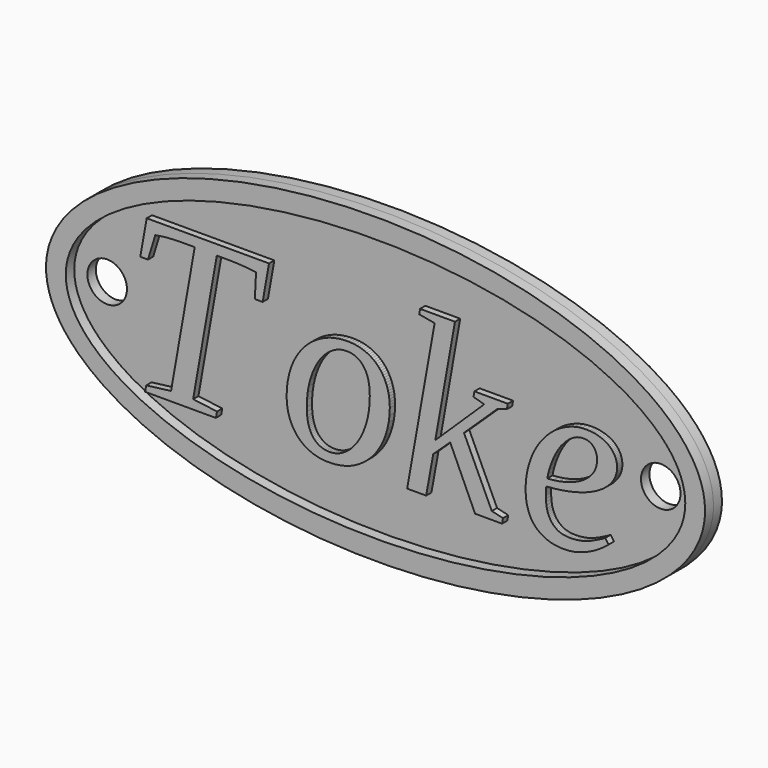
from build123d import *

# Parameters (mm, degrees)
F0_R     = 3
F1_DEPTH = 1.6
F2_DEPTH = 1.6
F3_DEPTH = 1


# Not quite as in the source:
# - a feature names something its author has since deleted; it is built from what else it names


with BuildPart() as f1:
    # F0 (on Front) → F1 (new body)
    with BuildSketch(Plane.XZ):
        with BuildLine():
            add(Edge.make_bspline(
                [(50, 0), (50, 39.8371685741), (-25, 19.918584287), (-100, 0), (-25, -19.918584287), (50, -39.8371685741), (50, 0)],
                knots=[0, 0, 0, 2.0943951024, 2.0943951024, 4.1887902048, 4.1887902048, 6.2831853072, 6.2831853072, 6.2831853072], degree=2, weights=[1, 0.5, 1, 0.5, 1, 0.5, 1]))
        make_face()
        with BuildLine():
            add(Edge.make_bspline(
                [(47, 0), (47, 34.6410161514), (-23.5, 17.3205080757), (-94, 0), (-23.5, -17.3205080757), (47, -34.6410161514), (47, 0)],
                knots=[0, 0, 0, 2.0943951024, 2.0943951024, 4.1887902048, 4.1887902048, 6.2831853072, 6.2831853072, 6.2831853072], degree=2, weights=[1, 0.5, 1, 0.5, 1, 0.5, 1]))
        make_face(mode=Mode.SUBTRACT)
        with BuildLine():
            add(Edge.make_bspline(
                [(47, 0), (47, 34.6410161514), (-23.5, 17.3205080757), (-94, 0), (-23.5, -17.3205080757), (47, -34.6410161514), (47, 0)],
                knots=[0, 0, 0, 2.0943951024, 2.0943951024, 4.1887902048, 4.1887902048, 6.2831853072, 6.2831853072, 6.2831853072], degree=2, weights=[1, 0.5, 1, 0.5, 1, 0.5, 1]))
        make_face()
        Polygon((-24.7064, -12.153), (-35.4455, -12.153), (-35.272, -11.2335), (-31.5072, -10.7651), (-27.916, 9.6201), (-28.8008, 9.6201), (-29.3451, 9.6179), (-29.8504, 9.6114), (-30.3166, 9.6006), (-30.5351, 9.5935), (-30.7439, 9.5854), (-31.1375, 9.5745), (-31.5029, 9.5594), (-31.8401, 9.5398), (-31.9982, 9.5284), (-32.1491, 9.516), (-32.4332, 9.4889), (-32.6956, 9.4596), (-32.8187, 9.4441), (-32.9364, 9.4281), (-33.0486, 9.4116), (-33.1554, 9.3945), (-33.3582, 9.3674), (-33.5501, 9.3382), (-33.7312, 9.3067), (-33.9014, 9.2731), (-35.0117, 5.6471), (-36.1741, 5.6471), (-35.2026, 11.1121), (-16.6391, 11.1121), (-17.6106, 5.6471), (-18.7904, 5.6471), (-18.6169, 9.2731), (-18.6952, 9.2881), (-18.7784, 9.3029), (-18.8665, 9.3174), (-18.9595, 9.3316), (-19.0574, 9.3456), (-19.1601, 9.3593), (-19.2677, 9.3727), (-19.4976, 9.3987), (-19.747, 9.4237), (-20.0159, 9.4475), (-20.3043, 9.4703), (-20.4559, 9.4813), (-20.7763, 9.5057), (-21.1216, 9.5268), (-21.4919, 9.5447), (-21.8872, 9.5594), (-22.3073, 9.5707), (-22.7525, 9.5789), (-23.2225, 9.5837), (-23.7175, 9.5854), (-24.5676, 9.5854), (-28.1589, -10.7651), (-24.5329, -11.2335), align=None, mode=Mode.SUBTRACT)
        Polygon((-7.0857, -12.487), (-7.6167, -12.5), (-7.9645, -12.4927), (-8.3052, -12.4707), (-8.6389, -12.4341), (-8.9656, -12.3829), (-9.2852, -12.317), (-9.5977, -12.2365), (-9.9033, -12.1413), (-10.2017, -12.0316), (-10.4874, -11.9079), (-10.7634, -11.7713), (-11.0296, -11.6217), (-11.286, -11.459), (-11.5327, -11.2834), (-11.7696, -11.0947), (-11.9968, -10.893), (-12.2142, -10.6783), (-12.4167, -10.4512), (-12.6078, -10.2121), (-12.7875, -9.9611), (-12.9559, -9.6981), (-13.1128, -9.4232), (-13.2584, -9.1364), (-13.3926, -8.8377), (-13.5154, -8.527), (-13.6211, -8.2053), (-13.7127, -7.8732), (-13.7903, -7.5308), (-13.8537, -7.1782), (-13.903, -6.8152), (-13.9383, -6.4419), (-13.9594, -6.0583), (-13.9665, -5.6645), (-13.9263, -4.6604), (-13.806, -3.678), (-13.6054, -2.7173), (-13.3245, -1.7783), (-13.1513, -1.3212), (-12.9613, -0.8783), (-12.7545, -0.4494), (-12.5308, -0.0347), (-12.2904, 0.366), (-12.0331, 0.7525), (-11.7591, 1.125), (-11.4682, 1.4834), (-11.1567, 1.8298), (-10.8295, 2.1578), (-10.4866, 2.4674), (-10.128, 2.7585), (-9.7536, 3.0312), (-9.3635, 3.2855), (-8.9577, 3.5213), (-8.5362, 3.7387), (-8.1, 3.938), (-7.6503, 4.1107), (-7.187, 4.2568), (-6.7102, 4.3763), (-6.2198, 4.4693), (-5.7159, 4.5357), (-5.1984, 4.5756), (-4.6674, 4.5888), (-4.3198, 4.5815), (-3.9799, 4.5596), (-3.6476, 4.523), (-3.3228, 4.4717), (-3.0056, 4.4059), (-2.6961, 4.3254), (-2.3941, 4.2302), (-2.0997, 4.1204), (-1.8102, 3.9968), (-1.5315, 3.8602), (-1.2637, 3.7105), (-1.0067, 3.5479), (-0.7606, 3.3722), (-0.5253, 3.1836), (-0.3008, 2.9819), (-0.0872, 2.7672), (0.1191, 2.54), (0.3129, 2.3009), (0.4943, 2.0499), (0.6631, 1.787), (0.8196, 1.5121), (0.9635, 1.2253), (1.095, 0.9266), (1.214, 0.6159), (1.3238, 0.2941), (1.4189, -0.0379), (1.4994, -0.3803), (1.5653, -0.733), (1.6165, -1.096), (1.6531, -1.4692), (1.6751, -1.8528), (1.6824, -2.2467), (1.6412, -3.2508), (1.5176, -4.2332), (1.3116, -5.1939), (1.0231, -6.1329), (0.8537, -6.5902), (0.6664, -7.0339), (0.4612, -7.4641), (0.2381, -7.8808), (-0.0029, -8.2839), (-0.2618, -8.6734), (-0.5386, -9.0494), (-0.8332, -9.4118), (-1.1406, -9.7545), (-1.4643, -10.0798), (-1.8042, -10.3877), (-2.1604, -10.6783), (-2.5329, -10.9516), (-2.9216, -11.2075), (-3.3266, -11.446), (-3.7479, -11.6672), (-4.184, -11.8624), (-4.6337, -12.0316), (-5.097, -12.1747), (-5.5739, -12.2918), (-6.0642, -12.3829), (-6.5682, -12.4479), align=None, mode=Mode.SUBTRACT)
        Polygon((36.1689, 1.2212), (36.1741, 1.0323), (36.163, 0.7523), (36.1296, 0.476), (36.074, 0.2036), (35.9962, -0.065), (35.8962, -0.3299), (35.774, -0.5909), (35.6295, -0.8482), (35.4628, -1.1016), (35.2746, -1.3502), (35.0659, -1.5928), (34.8366, -1.8295), (34.5866, -2.0602), (34.3161, -2.2849), (34.025, -2.5037), (33.7132, -2.7165), (33.3809, -2.9233), (33.0323, -3.119), (32.6631, -3.3071), (32.2732, -3.4877), (31.8628, -3.6606), (31.4318, -3.826), (30.9802, -3.9838), (30.0152, -4.2765), (28.9807, -4.5227), (27.8725, -4.7233), (26.6906, -4.8783), (25.435, -4.9878), (25.4328, -5.008), (25.4304, -5.0296), (25.4279, -5.0525), (25.4252, -5.0768), (25.4225, -5.1024), (25.4195, -5.1293), (25.4165, -5.1577), (25.4133, -5.1874), (25.4065, -5.2508), (25.3992, -5.3196), (25.3914, -5.3939), (25.383, -5.4736), (25.3789, -5.5579), (25.3724, -5.7379), (25.368, -5.9331), (25.3659, -6.1434), (25.3656, -6.2543), (25.3754, -6.6761), (25.4046, -7.0914), (25.4534, -7.5002), (25.5217, -7.9025), (25.5689, -8.0993), (25.6237, -8.2907), (25.686, -8.4766), (25.756, -8.6572), (25.8335, -8.8323), (25.9186, -9.002), (26.0113, -9.1662), (26.1116, -9.3251), (26.2203, -9.4774), (26.3382, -9.6222), (26.4654, -9.7594), (26.6017, -9.8889), (26.7473, -10.0109), (26.9021, -10.1253), (27.0661, -10.2321), (27.2393, -10.3313), (27.4231, -10.4167), (27.6188, -10.4907), (27.8265, -10.5534), (28.046, -10.6046), (28.2775, -10.6444), (28.521, -10.6729), (28.7763, -10.69), (29.0436, -10.6957), (29.4302, -10.6875), (29.8091, -10.6631), (30.1805, -10.6225), (30.5443, -10.5656), (30.9005, -10.4924), (31.2491, -10.4029), (31.5901, -10.2972), (31.9235, -10.1752), (32.572, -9.8976), (33.8038, -9.2904), (34.3871, -8.9608), (34.8902, -9.6894), (34.6007, -9.9258), (34.2874, -10.1665), (33.9501, -10.4116), (33.5891, -10.661), (33.2074, -10.9071), (32.8083, -11.1424), (31.9582, -11.5805), (31.518, -11.7713), (31.0648, -11.9448), (30.5985, -12.101), (30.1192, -12.2397), (29.6313, -12.3536), (29.139, -12.4349), (28.6424, -12.4837), (28.1415, -12.5), (27.7787, -12.4935), (27.428, -12.474), (27.0891, -12.4414), (26.7622, -12.3959), (26.4472, -12.3373), (26.1441, -12.2658), (25.853, -12.1812), (25.5738, -12.0836), (25.3062, -11.9697), (25.0501, -11.8451), (24.8053, -11.7095), (24.5719, -11.5631), (24.3499, -11.4059), (24.1392, -11.2378), (23.94, -11.0589), (23.7521, -10.8692), (23.5757, -10.6686), (23.4106, -10.4571), (23.2569, -10.2348), (23.1146, -10.0017), (22.9836, -9.7577), (22.8641, -9.5029), (22.7559, -9.2373), (22.6591, -8.9608), (22.5738, -8.6745), (22.4998, -8.3796), (22.4371, -8.076), (22.3859, -7.7637), (22.3461, -7.4427), (22.3005, -6.7748), (22.2948, -6.4278), (22.3165, -5.6645), (22.3816, -4.9184), (22.49, -4.1898), (22.6418, -3.4785), (22.8326, -2.7802), (23.0582, -2.1079), (23.3184, -1.4616), (23.6133, -0.8414), (23.9408, -0.2407), (24.2986, 0.3297), (24.6868, 0.8696), (25.1054, 1.3793), (25.5478, 1.864), (26.0075, 2.3118), (26.4846, 2.7227), (26.9791, 3.0968), (27.4974, 3.4319), (28.0287, 3.7257), (28.573, 3.9784), (29.1303, 4.1898), (29.705, 4.3644), (30.2841, 4.4891), (30.8674, 4.5639), (31.4551, 4.5888), (31.9951, 4.5715), (32.2537, 4.5498), (32.5047, 4.5194), (32.7482, 4.4804), (32.984, 4.4327), (33.2123, 4.3763), (33.4329, 4.3113), (33.6498, 4.2427), (33.858, 4.167), (34.0575, 4.0844), (34.2483, 3.9946), (34.4305, 3.8979), (34.604, 3.794), (34.7688, 3.6832), (34.9249, 3.5653), (35.0721, 3.4452), (35.2101, 3.3191), (35.3389, 3.1871), (35.4584, 3.0491), (35.5687, 2.9052), (35.6699, 2.7553), (35.7618, 2.5994), (35.8444, 2.4376), (35.9217, 2.2752), (35.9887, 2.109), (36.0453, 1.939), (36.0917, 1.7653), (36.1277, 1.5877), (36.1535, 1.4064), align=None, mode=Mode.SUBTRACT)
        with Locations((-42, 0)):
            Circle(F0_R, mode=Mode.SUBTRACT)
        Polygon((4.3203, -12.153), (8.4841, 11.3029), (6.142, 11.7193), (6.2808, 12.5), (11.5722, 12.5), (8.5882, -4.2939), (16.0136, 2.906), (14.3828, 3.3744), (14.5216, 4.1551), (19.5875, 4.1551), (19.4487, 3.3744), (18.0434, 2.9754), (12.9428, -1.8997), (17.1586, -10.9733), (18.8588, -11.3723), (18.72, -12.153), (14.6257, -12.153), (10.8436, -3.8428), (8.2759, -6.2543), (7.2003, -12.153), align=None, mode=Mode.SUBTRACT)
        with Locations((42, 0)):
            Circle(F0_R, mode=Mode.SUBTRACT)
        Polygon((-7.9645, -12.4927), (-7.6167, -12.5), (-7.0857, -12.487), (-6.5682, -12.4479), (-6.0642, -12.3829), (-5.5739, -12.2918), (-5.097, -12.1747), (-4.6337, -12.0316), (-4.184, -11.8624), (-3.7479, -11.6672), (-3.3266, -11.446), (-2.9216, -11.2075), (-2.5329, -10.9516), (-2.1604, -10.6783), (-1.8042, -10.3877), (-1.4643, -10.0798), (-1.1406, -9.7545), (-0.8332, -9.4118), (-0.5386, -9.0494), (-0.2618, -8.6734), (-0.0029, -8.2839), (0.2381, -7.8808), (0.4612, -7.4641), (0.6664, -7.0339), (0.8537, -6.5902), (1.0231, -6.1329), (1.3116, -5.1939), (1.5176, -4.2332), (1.6412, -3.2508), (1.6824, -2.2467), (1.6751, -1.8528), (1.6531, -1.4692), (1.6165, -1.096), (1.5653, -0.733), (1.4994, -0.3803), (1.4189, -0.0379), (1.3238, 0.2941), (1.214, 0.6159), (1.095, 0.9266), (0.9635, 1.2253), (0.8196, 1.5121), (0.6631, 1.787), (0.4943, 2.0499), (0.3129, 2.3009), (0.1191, 2.54), (-0.0872, 2.7672), (-0.3008, 2.9819), (-0.5253, 3.1836), (-0.7606, 3.3722), (-1.0067, 3.5479), (-1.2637, 3.7105), (-1.5315, 3.8602), (-1.8102, 3.9968), (-2.0997, 4.1204), (-2.3941, 4.2302), (-2.6961, 4.3254), (-3.0056, 4.4059), (-3.3228, 4.4717), (-3.6476, 4.523), (-3.9799, 4.5596), (-4.3198, 4.5815), (-4.6674, 4.5888), (-5.1984, 4.5756), (-5.7159, 4.5357), (-6.2198, 4.4693), (-6.7102, 4.3763), (-7.187, 4.2568), (-7.6503, 4.1107), (-8.1, 3.938), (-8.5362, 3.7387), (-8.9577, 3.5213), (-9.3635, 3.2855), (-9.7536, 3.0312), (-10.128, 2.7585), (-10.4866, 2.4674), (-10.8295, 2.1578), (-11.1567, 1.8298), (-11.4682, 1.4834), (-11.7591, 1.125), (-12.0331, 0.7525), (-12.2904, 0.366), (-12.5308, -0.0347), (-12.7545, -0.4494), (-12.9613, -0.8783), (-13.1513, -1.3212), (-13.3245, -1.7783), (-13.6054, -2.7173), (-13.806, -3.678), (-13.9263, -4.6604), (-13.9665, -5.6645), (-13.9594, -6.0583), (-13.9383, -6.4419), (-13.903, -6.8152), (-13.8537, -7.1782), (-13.7903, -7.5308), (-13.7127, -7.8732), (-13.6211, -8.2053), (-13.5154, -8.527), (-13.3926, -8.8377), (-13.2584, -9.1364), (-13.1128, -9.4232), (-12.9559, -9.6981), (-12.7875, -9.9611), (-12.6078, -10.2121), (-12.4167, -10.4512), (-12.2142, -10.6783), (-11.9968, -10.893), (-11.7696, -11.0947), (-11.5327, -11.2834), (-11.286, -11.459), (-11.0296, -11.6217), (-10.7634, -11.7713), (-10.4874, -11.9079), (-10.2017, -12.0316), (-9.9033, -12.1413), (-9.5977, -12.2365), (-9.2852, -12.317), (-8.9656, -12.3829), (-8.6389, -12.4341), (-8.3052, -12.4707), align=None)
        Polygon((-10.8989, -6.8228), (-10.913, -6.2543), (-10.8816, -5.2427), (-10.7872, -4.2722), (-10.63, -3.3429), (-10.4099, -2.4549), (-10.279, -2.0247), (-9.9862, -1.2114), (-9.8244, -0.8284), (-9.6522, -0.4611), (-9.4698, -0.1095), (-9.2771, 0.2264), (-9.074, 0.5465), (-8.8618, 0.8545), (-8.6414, 1.1451), (-8.4129, 1.4183), (-8.1762, 1.6742), (-7.9314, 1.9128), (-7.6785, 2.134), (-7.4175, 2.3378), (-7.1483, 2.5243), (-6.8737, 2.691), (-6.5964, 2.8355), (-6.3163, 2.9578), (-6.0336, 3.0578), (-5.7482, 3.1356), (-5.46, 3.1912), (-5.1691, 3.2245), (-4.8755, 3.2356), (-4.6661, 3.2307), (-4.463, 3.2161), (-4.266, 3.1917), (-4.0753, 3.1575), (-3.8909, 3.1136), (-3.7126, 3.06), (-3.5406, 2.9965), (-3.3749, 2.9233), (-3.2153, 2.8404), (-3.062, 2.7477), (-2.915, 2.6452), (-2.7741, 2.533), (-2.6396, 2.411), (-2.5112, 2.2793), (-2.3891, 2.1377), (-2.2732, 1.9865), (-2.1618, 1.828), (-2.0577, 1.6604), (-1.9607, 1.4837), (-1.8709, 1.2979), (-1.7883, 1.1031), (-1.7129, 0.8992), (-1.6446, 0.6862), (-1.5836, 0.4641), (-1.5297, 0.2329), (-1.483, -0.0073), (-1.4435, -0.2566), (-1.4112, -0.515), (-1.3681, -1.0591), (-1.3537, -1.6395), (-1.3862, -2.636), (-1.4838, -3.5956), (-1.6465, -4.5183), (-1.8742, -5.4042), (-2.0054, -5.8266), (-2.3003, -6.629), (-2.6386, -7.375), (-2.824, -7.7268), (-3.0203, -8.0646), (-3.2274, -8.3883), (-3.4399, -8.6924), (-3.6611, -8.9803), (-3.891, -9.2519), (-4.1295, -9.5073), (-4.3768, -9.7464), (-4.6327, -9.9692), (-4.8972, -10.1757), (-5.1705, -10.366), (-5.4454, -10.5328), (-5.7235, -10.6772), (-6.0049, -10.7995), (-6.2895, -10.8995), (-6.5774, -10.9773), (-6.8685, -11.0329), (-7.1629, -11.0662), (-7.4606, -11.0774), (-7.6616, -11.0725), (-7.8571, -11.0581), (-8.0471, -11.0341), (-8.2315, -11.0004), (-8.4104, -10.9571), (-8.5836, -10.9041), (-8.7514, -10.8416), (-8.9135, -10.7694), (-9.0702, -10.6876), (-9.2212, -10.5962), (-9.3667, -10.4951), (-9.5067, -10.3845), (-9.6411, -10.2642), (-9.7699, -10.1343), (-9.8932, -9.9947), (-10.0109, -9.8456), (-10.1201, -9.6852), (-10.2223, -9.5162), (-10.3175, -9.3387), (-10.4056, -9.1527), (-10.4866, -8.9581), (-10.5606, -8.755), (-10.6276, -8.5434), (-10.6875, -8.3232), (-10.7403, -8.0945), (-10.7862, -7.8572), (-10.8249, -7.6114), (-10.8566, -7.3571), align=None, mode=Mode.SUBTRACT)
        Polygon((36.163, 0.7523), (36.1741, 1.0323), (36.1689, 1.2212), (36.1535, 1.4064), (36.1277, 1.5877), (36.0917, 1.7653), (36.0453, 1.939), (35.9887, 2.109), (35.9217, 2.2752), (35.8444, 2.4376), (35.7618, 2.5994), (35.6699, 2.7553), (35.5687, 2.9052), (35.4584, 3.0491), (35.3389, 3.1871), (35.2101, 3.3191), (35.0721, 3.4452), (34.9249, 3.5653), (34.7688, 3.6832), (34.604, 3.794), (34.4305, 3.8979), (34.2483, 3.9946), (34.0575, 4.0844), (33.858, 4.167), (33.6498, 4.2427), (33.4329, 4.3113), (33.2123, 4.3763), (32.984, 4.4327), (32.7482, 4.4804), (32.5047, 4.5194), (32.2537, 4.5498), (31.9951, 4.5715), (31.4551, 4.5888), (30.8674, 4.5639), (30.2841, 4.4891), (29.705, 4.3644), (29.1303, 4.1898), (28.573, 3.9784), (28.0287, 3.7257), (27.4974, 3.4319), (26.9791, 3.0968), (26.4846, 2.7227), (26.0075, 2.3118), (25.5478, 1.864), (25.1054, 1.3793), (24.6868, 0.8696), (24.2986, 0.3297), (23.9408, -0.2407), (23.6133, -0.8414), (23.3184, -1.4616), (23.0582, -2.1079), (22.8326, -2.7802), (22.6418, -3.4785), (22.49, -4.1898), (22.3816, -4.9184), (22.3165, -5.6645), (22.2948, -6.4278), (22.3005, -6.7748), (22.3461, -7.4427), (22.3859, -7.7637), (22.4371, -8.076), (22.4998, -8.3796), (22.5738, -8.6745), (22.6591, -8.9608), (22.7559, -9.2373), (22.8641, -9.5029), (22.9836, -9.7577), (23.1146, -10.0017), (23.2569, -10.2348), (23.4106, -10.4571), (23.5757, -10.6686), (23.7521, -10.8692), (23.94, -11.0589), (24.1392, -11.2378), (24.3499, -11.4059), (24.5719, -11.5631), (24.8053, -11.7095), (25.0501, -11.8451), (25.3062, -11.9697), (25.5738, -12.0836), (25.853, -12.1812), (26.1441, -12.2658), (26.4472, -12.3373), (26.7622, -12.3959), (27.0891, -12.4414), (27.428, -12.474), (27.7787, -12.4935), (28.1415, -12.5), (28.6424, -12.4837), (29.139, -12.4349), (29.6313, -12.3536), (30.1192, -12.2397), (30.5985, -12.101), (31.0648, -11.9448), (31.518, -11.7713), (31.9582, -11.5805), (32.8083, -11.1424), (33.2074, -10.9071), (33.5891, -10.661), (33.9501, -10.4116), (34.2874, -10.1665), (34.6007, -9.9258), (34.8902, -9.6894), (34.3871, -8.9608), (33.8038, -9.2904), (32.572, -9.8976), (31.9235, -10.1752), (31.5901, -10.2972), (31.2491, -10.4029), (30.9005, -10.4924), (30.5443, -10.5656), (30.1805, -10.6225), (29.8091, -10.6631), (29.4302, -10.6875), (29.0436, -10.6957), (28.7763, -10.69), (28.521, -10.6729), (28.2775, -10.6444), (28.046, -10.6046), (27.8265, -10.5534), (27.6188, -10.4907), (27.4231, -10.4167), (27.2393, -10.3313), (27.0661, -10.2321), (26.9021, -10.1253), (26.7473, -10.0109), (26.6017, -9.8889), (26.4654, -9.7594), (26.3382, -9.6222), (26.2203, -9.4774), (26.1116, -9.3251), (26.0113, -9.1662), (25.9186, -9.002), (25.8335, -8.8323), (25.756, -8.6572), (25.686, -8.4766), (25.6237, -8.2907), (25.5689, -8.0993), (25.5217, -7.9025), (25.4534, -7.5002), (25.4046, -7.0914), (25.3754, -6.6761), (25.3656, -6.2543), (25.3659, -6.1434), (25.368, -5.9331), (25.3724, -5.7379), (25.3789, -5.5579), (25.383, -5.4736), (25.3914, -5.3939), (25.3992, -5.3196), (25.4065, -5.2508), (25.4133, -5.1874), (25.4165, -5.1577), (25.4195, -5.1293), (25.4225, -5.1024), (25.4252, -5.0768), (25.4279, -5.0525), (25.4304, -5.0296), (25.4328, -5.008), (25.435, -4.9878), (26.6906, -4.8783), (27.8725, -4.7233), (28.9807, -4.5227), (30.0152, -4.2765), (30.9802, -3.9838), (31.4318, -3.826), (31.8628, -3.6606), (32.2732, -3.4877), (32.6631, -3.3071), (33.0323, -3.119), (33.3809, -2.9233), (33.7132, -2.7165), (34.025, -2.5037), (34.3161, -2.2849), (34.5866, -2.0602), (34.8366, -1.8295), (35.0659, -1.5928), (35.2746, -1.3502), (35.4628, -1.1016), (35.6295, -0.8482), (35.774, -0.5909), (35.8962, -0.3299), (35.9962, -0.065), (36.074, 0.2036), (36.1296, 0.476), align=None)
        Polygon((26.49, -3.8059), (25.5738, -3.8948), (25.7039, -3.2692), (25.8687, -2.6414), (26.0682, -2.0114), (26.3025, -1.3792), (26.567, -0.7536), (26.8576, -0.1605), (27.1742, 0.4001), (27.5169, 0.9282), (27.7018, 1.1781), (28.0878, 1.6422), (28.2889, 1.8564), (28.4955, 2.0586), (28.7075, 2.2489), (28.9249, 2.4273), (29.1477, 2.5937), (29.3751, 2.7482), (29.6064, 2.8821), (29.8414, 2.9954), (30.0802, 3.0882), (30.3228, 3.1603), (30.5692, 3.2118), (30.8194, 3.2427), (31.0734, 3.253), (31.1973, 3.2505), (31.3174, 3.2432), (31.4337, 3.231), (31.5462, 3.2139), (31.6549, 3.192), (31.7598, 3.1651), (31.8609, 3.1334), (31.9582, 3.0968), (32.0518, 3.0553), (32.1415, 3.009), (32.2274, 2.9578), (32.3096, 2.9016), (32.3879, 2.8407), (32.4625, 2.7748), (32.5332, 2.704), (32.6002, 2.6284), (32.6653, 2.549), (32.7262, 2.4668), (32.7829, 2.382), (32.8355, 2.2944), (32.8838, 2.2042), (32.9279, 2.1112), (32.9678, 2.0155), (33.0035, 1.9171), (33.035, 1.816), (33.0624, 1.7122), (33.0855, 1.6056), (33.1044, 1.4964), (33.1191, 1.3844), (33.1296, 1.2698), (33.138, 1.0323), (33.1307, 0.8119), (33.1087, 0.5931), (33.0721, 0.376), (33.0209, 0.1605), (32.955, -0.0534), (32.8745, -0.2656), (32.7793, -0.4763), (32.6696, -0.6853), (32.5449, -0.887), (32.405, -1.0843), (32.2499, -1.2773), (32.0797, -1.466), (31.8943, -1.6503), (31.6937, -1.8303), (31.4779, -2.006), (31.2469, -2.1773), (31.0051, -2.3391), (30.7481, -2.495), (30.476, -2.6449), (30.1886, -2.7888), (29.8861, -2.9268), (29.5684, -3.0588), (29.2355, -3.1849), (28.8875, -3.305), (28.5245, -3.4129), (28.1469, -3.511), (27.3477, -3.678), align=None, mode=Mode.SUBTRACT)
        Polygon((6.142, 11.7193), (8.4841, 11.3029), (4.3203, -12.153), (7.2003, -12.153), (8.2759, -6.2543), (10.8436, -3.8428), (14.6257, -12.153), (18.72, -12.153), (18.8588, -11.3723), (17.1586, -10.9733), (12.9428, -1.8997), (18.0434, 2.9754), (19.4487, 3.3744), (19.5875, 4.1551), (14.5216, 4.1551), (14.3828, 3.3744), (16.0136, 2.906), (8.5882, -4.2939), (11.5722, 12.5), (6.2808, 12.5), align=None)
        Polygon((-35.272, -11.2335), (-35.4455, -12.153), (-24.7064, -12.153), (-24.5329, -11.2335), (-28.1589, -10.7651), (-24.5676, 9.5854), (-23.7175, 9.5854), (-23.2225, 9.5837), (-22.7525, 9.5789), (-22.3073, 9.5707), (-21.8872, 9.5594), (-21.4919, 9.5447), (-21.1216, 9.5268), (-20.7763, 9.5057), (-20.4559, 9.4813), (-20.3043, 9.4703), (-20.0159, 9.4475), (-19.747, 9.4237), (-19.4976, 9.3987), (-19.2677, 9.3727), (-19.1601, 9.3593), (-19.0574, 9.3456), (-18.9595, 9.3316), (-18.8665, 9.3174), (-18.7784, 9.3029), (-18.6952, 9.2881), (-18.6169, 9.2731), (-18.7904, 5.6471), (-17.6106, 5.6471), (-16.6391, 11.1121), (-35.2026, 11.1121), (-36.1741, 5.6471), (-35.0117, 5.6471), (-33.9014, 9.2731), (-33.7312, 9.3067), (-33.5501, 9.3382), (-33.3582, 9.3674), (-33.1554, 9.3945), (-33.0486, 9.4116), (-32.9364, 9.4281), (-32.8187, 9.4441), (-32.6956, 9.4596), (-32.4332, 9.4889), (-32.1491, 9.516), (-31.9982, 9.5284), (-31.8401, 9.5398), (-31.5029, 9.5594), (-31.1375, 9.5745), (-30.7439, 9.5854), (-30.5351, 9.5935), (-30.3166, 9.6006), (-29.8504, 9.6114), (-29.3451, 9.6179), (-28.8008, 9.6201), (-27.916, 9.6201), (-31.5072, -10.7651), align=None)
        Polygon((-10.8816, -5.2427), (-10.913, -6.2543), (-10.8989, -6.8228), (-10.8566, -7.3571), (-10.8249, -7.6114), (-10.7862, -7.8572), (-10.7403, -8.0945), (-10.6875, -8.3232), (-10.6276, -8.5434), (-10.5606, -8.755), (-10.4866, -8.9581), (-10.4056, -9.1527), (-10.3175, -9.3387), (-10.2223, -9.5162), (-10.1201, -9.6852), (-10.0109, -9.8456), (-9.8932, -9.9947), (-9.7699, -10.1343), (-9.6411, -10.2642), (-9.5067, -10.3845), (-9.3667, -10.4951), (-9.2212, -10.5962), (-9.0702, -10.6876), (-8.9135, -10.7694), (-8.7514, -10.8416), (-8.5836, -10.9041), (-8.4104, -10.9571), (-8.2315, -11.0004), (-8.0471, -11.0341), (-7.8571, -11.0581), (-7.6616, -11.0725), (-7.4606, -11.0774), (-7.1629, -11.0662), (-6.8685, -11.0329), (-6.5774, -10.9773), (-6.2895, -10.8995), (-6.0049, -10.7995), (-5.7235, -10.6772), (-5.4454, -10.5328), (-5.1705, -10.366), (-4.8972, -10.1757), (-4.6327, -9.9692), (-4.3768, -9.7464), (-4.1295, -9.5073), (-3.891, -9.2519), (-3.6611, -8.9803), (-3.4399, -8.6924), (-3.2274, -8.3883), (-3.0203, -8.0646), (-2.824, -7.7268), (-2.6386, -7.375), (-2.3003, -6.629), (-2.0054, -5.8266), (-1.8742, -5.4042), (-1.6465, -4.5183), (-1.4838, -3.5956), (-1.3862, -2.636), (-1.3537, -1.6395), (-1.3681, -1.0591), (-1.4112, -0.515), (-1.4435, -0.2566), (-1.483, -0.0073), (-1.5297, 0.2329), (-1.5836, 0.4641), (-1.6446, 0.6862), (-1.7129, 0.8992), (-1.7883, 1.1031), (-1.8709, 1.2979), (-1.9607, 1.4837), (-2.0577, 1.6604), (-2.1618, 1.828), (-2.2732, 1.9865), (-2.3891, 2.1377), (-2.5112, 2.2793), (-2.6396, 2.411), (-2.7741, 2.533), (-2.915, 2.6452), (-3.062, 2.7477), (-3.2153, 2.8404), (-3.3749, 2.9233), (-3.5406, 2.9965), (-3.7126, 3.06), (-3.8909, 3.1136), (-4.0753, 3.1575), (-4.266, 3.1917), (-4.463, 3.2161), (-4.6661, 3.2307), (-4.8755, 3.2356), (-5.1691, 3.2245), (-5.46, 3.1912), (-5.7482, 3.1356), (-6.0336, 3.0578), (-6.3163, 2.9578), (-6.5964, 2.8355), (-6.8737, 2.691), (-7.1483, 2.5243), (-7.4175, 2.3378), (-7.6785, 2.134), (-7.9314, 1.9128), (-8.1762, 1.6742), (-8.4129, 1.4183), (-8.6414, 1.1451), (-8.8618, 0.8545), (-9.074, 0.5465), (-9.2771, 0.2264), (-9.4698, -0.1095), (-9.6522, -0.4611), (-9.8244, -0.8284), (-9.9862, -1.2114), (-10.279, -2.0247), (-10.4099, -2.4549), (-10.63, -3.3429), (-10.7872, -4.2722), align=None)
        Polygon((25.7039, -3.2692), (25.5738, -3.8948), (26.49, -3.8059), (27.3477, -3.678), (28.1469, -3.511), (28.5245, -3.4129), (28.8875, -3.305), (29.2355, -3.1849), (29.5684, -3.0588), (29.8861, -2.9268), (30.1886, -2.7888), (30.476, -2.6449), (30.7481, -2.495), (31.0051, -2.3391), (31.2469, -2.1773), (31.4779, -2.006), (31.6937, -1.8303), (31.8943, -1.6503), (32.0797, -1.466), (32.2499, -1.2773), (32.405, -1.0843), (32.5449, -0.887), (32.6696, -0.6853), (32.7793, -0.4763), (32.8745, -0.2656), (32.955, -0.0534), (33.0209, 0.1605), (33.0721, 0.376), (33.1087, 0.5931), (33.1307, 0.8119), (33.138, 1.0323), (33.1296, 1.2698), (33.1191, 1.3844), (33.1044, 1.4964), (33.0855, 1.6056), (33.0624, 1.7122), (33.035, 1.816), (33.0035, 1.9171), (32.9678, 2.0155), (32.9279, 2.1112), (32.8838, 2.2042), (32.8355, 2.2944), (32.7829, 2.382), (32.7262, 2.4668), (32.6653, 2.549), (32.6002, 2.6284), (32.5332, 2.704), (32.4625, 2.7748), (32.3879, 2.8407), (32.3096, 2.9016), (32.2274, 2.9578), (32.1415, 3.009), (32.0518, 3.0553), (31.9582, 3.0968), (31.8609, 3.1334), (31.7598, 3.1651), (31.6549, 3.192), (31.5462, 3.2139), (31.4337, 3.231), (31.3174, 3.2432), (31.1973, 3.2505), (31.0734, 3.253), (30.8194, 3.2427), (30.5692, 3.2118), (30.3228, 3.1603), (30.0802, 3.0882), (29.8414, 2.9954), (29.6064, 2.8821), (29.3751, 2.7482), (29.1477, 2.5937), (28.9249, 2.4273), (28.7075, 2.2489), (28.4955, 2.0586), (28.2889, 1.8564), (28.0878, 1.6422), (27.7018, 1.1781), (27.5169, 0.9282), (27.1742, 0.4001), (26.8576, -0.1605), (26.567, -0.7536), (26.3025, -1.3792), (26.0682, -2.0114), (25.8687, -2.6414), align=None)
    extrude(amount=-F1_DEPTH)

    # F0 (on Front) → F2 (join)
    with BuildSketch(Plane.XZ):
        with BuildLine():
            add(Edge.make_bspline(
                [(50, 0), (50, 39.8371685741), (-25, 19.918584287), (-100, 0), (-25, -19.918584287), (50, -39.8371685741), (50, 0)],
                knots=[0, 0, 0, 2.0943951024, 2.0943951024, 4.1887902048, 4.1887902048, 6.2831853072, 6.2831853072, 6.2831853072], degree=2, weights=[1, 0.5, 1, 0.5, 1, 0.5, 1]))
        make_face()
        with BuildLine():
            add(Edge.make_bspline(
                [(47, 0), (47, 34.6410161514), (-23.5, 17.3205080757), (-94, 0), (-23.5, -17.3205080757), (47, -34.6410161514), (47, 0)],
                knots=[0, 0, 0, 2.0943951024, 2.0943951024, 4.1887902048, 4.1887902048, 6.2831853072, 6.2831853072, 6.2831853072], degree=2, weights=[1, 0.5, 1, 0.5, 1, 0.5, 1]))
        make_face(mode=Mode.SUBTRACT)
    extrude(amount=F2_DEPTH)

    # F0 (on Front) → F3 (join)
    with BuildSketch(Plane.XZ):
        Polygon((-7.9645, -12.4927), (-7.6167, -12.5), (-7.0857, -12.487), (-6.5682, -12.4479), (-6.0642, -12.3829), (-5.5739, -12.2918), (-5.097, -12.1747), (-4.6337, -12.0316), (-4.184, -11.8624), (-3.7479, -11.6672), (-3.3266, -11.446), (-2.9216, -11.2075), (-2.5329, -10.9516), (-2.1604, -10.6783), (-1.8042, -10.3877), (-1.4643, -10.0798), (-1.1406, -9.7545), (-0.8332, -9.4118), (-0.5386, -9.0494), (-0.2618, -8.6734), (-0.0029, -8.2839), (0.2381, -7.8808), (0.4612, -7.4641), (0.6664, -7.0339), (0.8537, -6.5902), (1.0231, -6.1329), (1.3116, -5.1939), (1.5176, -4.2332), (1.6412, -3.2508), (1.6824, -2.2467), (1.6751, -1.8528), (1.6531, -1.4692), (1.6165, -1.096), (1.5653, -0.733), (1.4994, -0.3803), (1.4189, -0.0379), (1.3238, 0.2941), (1.214, 0.6159), (1.095, 0.9266), (0.9635, 1.2253), (0.8196, 1.5121), (0.6631, 1.787), (0.4943, 2.0499), (0.3129, 2.3009), (0.1191, 2.54), (-0.0872, 2.7672), (-0.3008, 2.9819), (-0.5253, 3.1836), (-0.7606, 3.3722), (-1.0067, 3.5479), (-1.2637, 3.7105), (-1.5315, 3.8602), (-1.8102, 3.9968), (-2.0997, 4.1204), (-2.3941, 4.2302), (-2.6961, 4.3254), (-3.0056, 4.4059), (-3.3228, 4.4717), (-3.6476, 4.523), (-3.9799, 4.5596), (-4.3198, 4.5815), (-4.6674, 4.5888), (-5.1984, 4.5756), (-5.7159, 4.5357), (-6.2198, 4.4693), (-6.7102, 4.3763), (-7.187, 4.2568), (-7.6503, 4.1107), (-8.1, 3.938), (-8.5362, 3.7387), (-8.9577, 3.5213), (-9.3635, 3.2855), (-9.7536, 3.0312), (-10.128, 2.7585), (-10.4866, 2.4674), (-10.8295, 2.1578), (-11.1567, 1.8298), (-11.4682, 1.4834), (-11.7591, 1.125), (-12.0331, 0.7525), (-12.2904, 0.366), (-12.5308, -0.0347), (-12.7545, -0.4494), (-12.9613, -0.8783), (-13.1513, -1.3212), (-13.3245, -1.7783), (-13.6054, -2.7173), (-13.806, -3.678), (-13.9263, -4.6604), (-13.9665, -5.6645), (-13.9594, -6.0583), (-13.9383, -6.4419), (-13.903, -6.8152), (-13.8537, -7.1782), (-13.7903, -7.5308), (-13.7127, -7.8732), (-13.6211, -8.2053), (-13.5154, -8.527), (-13.3926, -8.8377), (-13.2584, -9.1364), (-13.1128, -9.4232), (-12.9559, -9.6981), (-12.7875, -9.9611), (-12.6078, -10.2121), (-12.4167, -10.4512), (-12.2142, -10.6783), (-11.9968, -10.893), (-11.7696, -11.0947), (-11.5327, -11.2834), (-11.286, -11.459), (-11.0296, -11.6217), (-10.7634, -11.7713), (-10.4874, -11.9079), (-10.2017, -12.0316), (-9.9033, -12.1413), (-9.5977, -12.2365), (-9.2852, -12.317), (-8.9656, -12.3829), (-8.6389, -12.4341), (-8.3052, -12.4707), align=None)
        Polygon((-10.8989, -6.8228), (-10.913, -6.2543), (-10.8816, -5.2427), (-10.7872, -4.2722), (-10.63, -3.3429), (-10.4099, -2.4549), (-10.279, -2.0247), (-9.9862, -1.2114), (-9.8244, -0.8284), (-9.6522, -0.4611), (-9.4698, -0.1095), (-9.2771, 0.2264), (-9.074, 0.5465), (-8.8618, 0.8545), (-8.6414, 1.1451), (-8.4129, 1.4183), (-8.1762, 1.6742), (-7.9314, 1.9128), (-7.6785, 2.134), (-7.4175, 2.3378), (-7.1483, 2.5243), (-6.8737, 2.691), (-6.5964, 2.8355), (-6.3163, 2.9578), (-6.0336, 3.0578), (-5.7482, 3.1356), (-5.46, 3.1912), (-5.1691, 3.2245), (-4.8755, 3.2356), (-4.6661, 3.2307), (-4.463, 3.2161), (-4.266, 3.1917), (-4.0753, 3.1575), (-3.8909, 3.1136), (-3.7126, 3.06), (-3.5406, 2.9965), (-3.3749, 2.9233), (-3.2153, 2.8404), (-3.062, 2.7477), (-2.915, 2.6452), (-2.7741, 2.533), (-2.6396, 2.411), (-2.5112, 2.2793), (-2.3891, 2.1377), (-2.2732, 1.9865), (-2.1618, 1.828), (-2.0577, 1.6604), (-1.9607, 1.4837), (-1.8709, 1.2979), (-1.7883, 1.1031), (-1.7129, 0.8992), (-1.6446, 0.6862), (-1.5836, 0.4641), (-1.5297, 0.2329), (-1.483, -0.0073), (-1.4435, -0.2566), (-1.4112, -0.515), (-1.3681, -1.0591), (-1.3537, -1.6395), (-1.3862, -2.636), (-1.4838, -3.5956), (-1.6465, -4.5183), (-1.8742, -5.4042), (-2.0054, -5.8266), (-2.3003, -6.629), (-2.6386, -7.375), (-2.824, -7.7268), (-3.0203, -8.0646), (-3.2274, -8.3883), (-3.4399, -8.6924), (-3.6611, -8.9803), (-3.891, -9.2519), (-4.1295, -9.5073), (-4.3768, -9.7464), (-4.6327, -9.9692), (-4.8972, -10.1757), (-5.1705, -10.366), (-5.4454, -10.5328), (-5.7235, -10.6772), (-6.0049, -10.7995), (-6.2895, -10.8995), (-6.5774, -10.9773), (-6.8685, -11.0329), (-7.1629, -11.0662), (-7.4606, -11.0774), (-7.6616, -11.0725), (-7.8571, -11.0581), (-8.0471, -11.0341), (-8.2315, -11.0004), (-8.4104, -10.9571), (-8.5836, -10.9041), (-8.7514, -10.8416), (-8.9135, -10.7694), (-9.0702, -10.6876), (-9.2212, -10.5962), (-9.3667, -10.4951), (-9.5067, -10.3845), (-9.6411, -10.2642), (-9.7699, -10.1343), (-9.8932, -9.9947), (-10.0109, -9.8456), (-10.1201, -9.6852), (-10.2223, -9.5162), (-10.3175, -9.3387), (-10.4056, -9.1527), (-10.4866, -8.9581), (-10.5606, -8.755), (-10.6276, -8.5434), (-10.6875, -8.3232), (-10.7403, -8.0945), (-10.7862, -7.8572), (-10.8249, -7.6114), (-10.8566, -7.3571), align=None, mode=Mode.SUBTRACT)
        Polygon((6.142, 11.7193), (8.4841, 11.3029), (4.3203, -12.153), (7.2003, -12.153), (8.2759, -6.2543), (10.8436, -3.8428), (14.6257, -12.153), (18.72, -12.153), (18.8588, -11.3723), (17.1586, -10.9733), (12.9428, -1.8997), (18.0434, 2.9754), (19.4487, 3.3744), (19.5875, 4.1551), (14.5216, 4.1551), (14.3828, 3.3744), (16.0136, 2.906), (8.5882, -4.2939), (11.5722, 12.5), (6.2808, 12.5), align=None)
        Polygon((36.163, 0.7523), (36.1741, 1.0323), (36.1689, 1.2212), (36.1535, 1.4064), (36.1277, 1.5877), (36.0917, 1.7653), (36.0453, 1.939), (35.9887, 2.109), (35.9217, 2.2752), (35.8444, 2.4376), (35.7618, 2.5994), (35.6699, 2.7553), (35.5687, 2.9052), (35.4584, 3.0491), (35.3389, 3.1871), (35.2101, 3.3191), (35.0721, 3.4452), (34.9249, 3.5653), (34.7688, 3.6832), (34.604, 3.794), (34.4305, 3.8979), (34.2483, 3.9946), (34.0575, 4.0844), (33.858, 4.167), (33.6498, 4.2427), (33.4329, 4.3113), (33.2123, 4.3763), (32.984, 4.4327), (32.7482, 4.4804), (32.5047, 4.5194), (32.2537, 4.5498), (31.9951, 4.5715), (31.4551, 4.5888), (30.8674, 4.5639), (30.2841, 4.4891), (29.705, 4.3644), (29.1303, 4.1898), (28.573, 3.9784), (28.0287, 3.7257), (27.4974, 3.4319), (26.9791, 3.0968), (26.4846, 2.7227), (26.0075, 2.3118), (25.5478, 1.864), (25.1054, 1.3793), (24.6868, 0.8696), (24.2986, 0.3297), (23.9408, -0.2407), (23.6133, -0.8414), (23.3184, -1.4616), (23.0582, -2.1079), (22.8326, -2.7802), (22.6418, -3.4785), (22.49, -4.1898), (22.3816, -4.9184), (22.3165, -5.6645), (22.2948, -6.4278), (22.3005, -6.7748), (22.3461, -7.4427), (22.3859, -7.7637), (22.4371, -8.076), (22.4998, -8.3796), (22.5738, -8.6745), (22.6591, -8.9608), (22.7559, -9.2373), (22.8641, -9.5029), (22.9836, -9.7577), (23.1146, -10.0017), (23.2569, -10.2348), (23.4106, -10.4571), (23.5757, -10.6686), (23.7521, -10.8692), (23.94, -11.0589), (24.1392, -11.2378), (24.3499, -11.4059), (24.5719, -11.5631), (24.8053, -11.7095), (25.0501, -11.8451), (25.3062, -11.9697), (25.5738, -12.0836), (25.853, -12.1812), (26.1441, -12.2658), (26.4472, -12.3373), (26.7622, -12.3959), (27.0891, -12.4414), (27.428, -12.474), (27.7787, -12.4935), (28.1415, -12.5), (28.6424, -12.4837), (29.139, -12.4349), (29.6313, -12.3536), (30.1192, -12.2397), (30.5985, -12.101), (31.0648, -11.9448), (31.518, -11.7713), (31.9582, -11.5805), (32.8083, -11.1424), (33.2074, -10.9071), (33.5891, -10.661), (33.9501, -10.4116), (34.2874, -10.1665), (34.6007, -9.9258), (34.8902, -9.6894), (34.3871, -8.9608), (33.8038, -9.2904), (32.572, -9.8976), (31.9235, -10.1752), (31.5901, -10.2972), (31.2491, -10.4029), (30.9005, -10.4924), (30.5443, -10.5656), (30.1805, -10.6225), (29.8091, -10.6631), (29.4302, -10.6875), (29.0436, -10.6957), (28.7763, -10.69), (28.521, -10.6729), (28.2775, -10.6444), (28.046, -10.6046), (27.8265, -10.5534), (27.6188, -10.4907), (27.4231, -10.4167), (27.2393, -10.3313), (27.0661, -10.2321), (26.9021, -10.1253), (26.7473, -10.0109), (26.6017, -9.8889), (26.4654, -9.7594), (26.3382, -9.6222), (26.2203, -9.4774), (26.1116, -9.3251), (26.0113, -9.1662), (25.9186, -9.002), (25.8335, -8.8323), (25.756, -8.6572), (25.686, -8.4766), (25.6237, -8.2907), (25.5689, -8.0993), (25.5217, -7.9025), (25.4534, -7.5002), (25.4046, -7.0914), (25.3754, -6.6761), (25.3656, -6.2543), (25.3659, -6.1434), (25.368, -5.9331), (25.3724, -5.7379), (25.3789, -5.5579), (25.383, -5.4736), (25.3914, -5.3939), (25.3992, -5.3196), (25.4065, -5.2508), (25.4133, -5.1874), (25.4165, -5.1577), (25.4195, -5.1293), (25.4225, -5.1024), (25.4252, -5.0768), (25.4279, -5.0525), (25.4304, -5.0296), (25.4328, -5.008), (25.435, -4.9878), (26.6906, -4.8783), (27.8725, -4.7233), (28.9807, -4.5227), (30.0152, -4.2765), (30.9802, -3.9838), (31.4318, -3.826), (31.8628, -3.6606), (32.2732, -3.4877), (32.6631, -3.3071), (33.0323, -3.119), (33.3809, -2.9233), (33.7132, -2.7165), (34.025, -2.5037), (34.3161, -2.2849), (34.5866, -2.0602), (34.8366, -1.8295), (35.0659, -1.5928), (35.2746, -1.3502), (35.4628, -1.1016), (35.6295, -0.8482), (35.774, -0.5909), (35.8962, -0.3299), (35.9962, -0.065), (36.074, 0.2036), (36.1296, 0.476), align=None)
        Polygon((26.49, -3.8059), (25.5738, -3.8948), (25.7039, -3.2692), (25.8687, -2.6414), (26.0682, -2.0114), (26.3025, -1.3792), (26.567, -0.7536), (26.8576, -0.1605), (27.1742, 0.4001), (27.5169, 0.9282), (27.7018, 1.1781), (28.0878, 1.6422), (28.2889, 1.8564), (28.4955, 2.0586), (28.7075, 2.2489), (28.9249, 2.4273), (29.1477, 2.5937), (29.3751, 2.7482), (29.6064, 2.8821), (29.8414, 2.9954), (30.0802, 3.0882), (30.3228, 3.1603), (30.5692, 3.2118), (30.8194, 3.2427), (31.0734, 3.253), (31.1973, 3.2505), (31.3174, 3.2432), (31.4337, 3.231), (31.5462, 3.2139), (31.6549, 3.192), (31.7598, 3.1651), (31.8609, 3.1334), (31.9582, 3.0968), (32.0518, 3.0553), (32.1415, 3.009), (32.2274, 2.9578), (32.3096, 2.9016), (32.3879, 2.8407), (32.4625, 2.7748), (32.5332, 2.704), (32.6002, 2.6284), (32.6653, 2.549), (32.7262, 2.4668), (32.7829, 2.382), (32.8355, 2.2944), (32.8838, 2.2042), (32.9279, 2.1112), (32.9678, 2.0155), (33.0035, 1.9171), (33.035, 1.816), (33.0624, 1.7122), (33.0855, 1.6056), (33.1044, 1.4964), (33.1191, 1.3844), (33.1296, 1.2698), (33.138, 1.0323), (33.1307, 0.8119), (33.1087, 0.5931), (33.0721, 0.376), (33.0209, 0.1605), (32.955, -0.0534), (32.8745, -0.2656), (32.7793, -0.4763), (32.6696, -0.6853), (32.5449, -0.887), (32.405, -1.0843), (32.2499, -1.2773), (32.0797, -1.466), (31.8943, -1.6503), (31.6937, -1.8303), (31.4779, -2.006), (31.2469, -2.1773), (31.0051, -2.3391), (30.7481, -2.495), (30.476, -2.6449), (30.1886, -2.7888), (29.8861, -2.9268), (29.5684, -3.0588), (29.2355, -3.1849), (28.8875, -3.305), (28.5245, -3.4129), (28.1469, -3.511), (27.3477, -3.678), align=None, mode=Mode.SUBTRACT)
        Polygon((-35.272, -11.2335), (-35.4455, -12.153), (-24.7064, -12.153), (-24.5329, -11.2335), (-28.1589, -10.7651), (-24.5676, 9.5854), (-23.7175, 9.5854), (-23.2225, 9.5837), (-22.7525, 9.5789), (-22.3073, 9.5707), (-21.8872, 9.5594), (-21.4919, 9.5447), (-21.1216, 9.5268), (-20.7763, 9.5057), (-20.4559, 9.4813), (-20.3043, 9.4703), (-20.0159, 9.4475), (-19.747, 9.4237), (-19.4976, 9.3987), (-19.2677, 9.3727), (-19.1601, 9.3593), (-19.0574, 9.3456), (-18.9595, 9.3316), (-18.8665, 9.3174), (-18.7784, 9.3029), (-18.6952, 9.2881), (-18.6169, 9.2731), (-18.7904, 5.6471), (-17.6106, 5.6471), (-16.6391, 11.1121), (-35.2026, 11.1121), (-36.1741, 5.6471), (-35.0117, 5.6471), (-33.9014, 9.2731), (-33.7312, 9.3067), (-33.5501, 9.3382), (-33.3582, 9.3674), (-33.1554, 9.3945), (-33.0486, 9.4116), (-32.9364, 9.4281), (-32.8187, 9.4441), (-32.6956, 9.4596), (-32.4332, 9.4889), (-32.1491, 9.516), (-31.9982, 9.5284), (-31.8401, 9.5398), (-31.5029, 9.5594), (-31.1375, 9.5745), (-30.7439, 9.5854), (-30.5351, 9.5935), (-30.3166, 9.6006), (-29.8504, 9.6114), (-29.3451, 9.6179), (-28.8008, 9.6201), (-27.916, 9.6201), (-31.5072, -10.7651), align=None)
    extrude(amount=F3_DEPTH)


solid = f1.part
